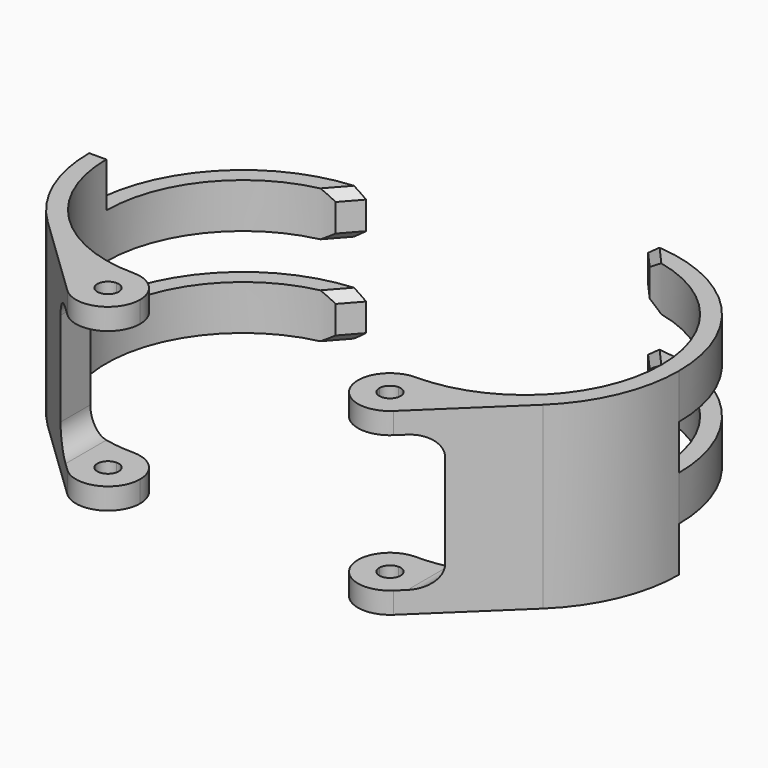
from build123d import *

# Parameters (mm, degrees)
F1_DEPTH      = 21
F2_W          = 90
F2_H          = 32
F3_DEPTH      = 60
F4_R          = 5
F4_2_R        = 5
F5_W          = 36
F5_H          = 10.5
F6_DEPTH      = 80
F7_W          = 36
F7_H          = 10.5
F8_DEPTH      = 80
F9_T1_DEPTH   = 31.1430234422
F9_T3_DEPTH   = 31.1430234422
F9_2_T1_DEPTH = 31.1430234422
F9_2_T3_DEPTH = 31.1430234422
F10_SIZE      = 2
F10_2_SIZE    = 2


# Not quite as in the source:
# - a fillet or chamfer that OpenCascade refuses, or shapes differently, is made with other operations: its cross-section is extruded or revolved along the edge and cut away or added


with BuildPart() as f1:
    # F0 (on Top) → F1 (new body, symmetric)
    with BuildSketch(Plane.XY):
        with BuildLine():
            ThreePointArc((-33, -32), (-65, 0), (-33, 32))
            Line((-33, 32), (-33, 36))
            ThreePointArc((-33, 36), (-66.3997650261, 13.4333799247), (-57.9262073885, -25.9746835443))
            ThreePointArc((-57.9262073885, -25.9746835443), (-49.3189032488, -32.0888360144), (-39.3080154665, -35.4430379747))
            ThreePointArc((-39.3080154665, -35.4430379747), (-36.5932426031, -32.9167935172), (-33, -32))
        make_face()
        with BuildLine():
            Line((-33, -36), (-33, -32))
            ThreePointArc((-33, -32), (-36.5932426031, -32.9167935172), (-39.3080154665, -35.4430379747))
            ThreePointArc((-39.3080154665, -35.4430379747), (-36.166278013, -35.8604891705), (-33, -36))
        make_face()
        with BuildLine():
            ThreePointArc((-26.6919845335, -35.4430379747), (-29.4067573969, -32.9167935172), (-33, -32))
            Line((-33, -32), (-33, -36))
            ThreePointArc((-33, -36), (-29.833721987, -35.8604891705), (-26.6919845335, -35.4430379747))
        make_face()
        with BuildLine():
            ThreePointArc((-25.5, -39.5), (-25.8041638429, -37.3857762652), (-26.6919845335, -35.4430379747))
            ThreePointArc((-26.6919845335, -35.4430379747), (-29.833721987, -35.8604891705), (-33, -36))
            Line((-33, -36), (-33, -37))
            ThreePointArc((-33, -37), (-31.232233047, -37.732233047), (-30.5, -39.5))
            Line((-30.5, -39.5), (-25.5, -39.5))
        make_face()
        with BuildLine():
            ThreePointArc((-38.1929598726, -44.9113924051), (-40.4485261859, -40.3771873561), (-39.3080154665, -35.4430379747))
            ThreePointArc((-39.3080154665, -35.4430379747), (-49.3189032488, -32.0888360144), (-57.9262073885, -25.9746835443))
            Line((-57.9262073885, -25.9746835443), (-38.1929598726, -44.9113924051))
        make_face()
        with BuildLine():
            ThreePointArc((-33, -36), (-36.166278013, -35.8604891705), (-39.3080154665, -35.4430379747))
            ThreePointArc((-39.3080154665, -35.4430379747), (-40.4485261859, -40.3771873561), (-38.1929598726, -44.9113924051))
            ThreePointArc((-38.1929598726, -44.9113924051), (-30.0586736873, -46.399173829), (-25.5, -39.5))
            Line((-25.5, -39.5), (-30.5, -39.5))
            ThreePointArc((-30.5, -39.5), (-34.767766953, -41.267766953), (-33, -37))
            Line((-33, -37), (-33, -36))
        make_face()
    extrude(amount=F1_DEPTH, both=True)


with BuildPart() as f1b:
    # F0 (on Top) → F1, piece 2 (new body, symmetric)
    with BuildSketch(Plane.XY):
        with BuildLine():
            ThreePointArc((69, 0), (58.4558441227, 25.4558441227), (33, 36))
            Line((33, 36), (33, 32))
            ThreePointArc((33, 32), (55.627416998, 22.627416998), (65, 0))
            ThreePointArc((65, 0), (55.627416998, -22.627416998), (33, -32))
            ThreePointArc((33, -32), (36.5932426031, -32.9167935172), (39.3080154665, -35.4430379747))
            ThreePointArc((39.3080154665, -35.4430379747), (49.3189032488, -32.0888360144), (57.9262073885, -25.9746835443))
            ThreePointArc((57.9262073885, -25.9746835443), (66.116034379, -14.1183663009), (69, 0))
        make_face()
        with BuildLine():
            ThreePointArc((33, -32), (29.4067573969, -32.9167935172), (26.6919845335, -35.4430379747))
            ThreePointArc((26.6919845335, -35.4430379747), (29.833721987, -35.8604891705), (33, -36))
            Line((33, -36), (33, -32))
        make_face()
        with BuildLine():
            ThreePointArc((33, -36), (29.833721987, -35.8604891705), (26.6919845335, -35.4430379747))
            ThreePointArc((26.6919845335, -35.4430379747), (25.8041638429, -37.3857762652), (25.5, -39.5))
            Line((25.5, -39.5), (30.5, -39.5))
            ThreePointArc((30.5, -39.5), (31.232233047, -37.732233047), (33, -37))
            Line((33, -37), (33, -36))
        make_face()
        with BuildLine():
            ThreePointArc((39.3080154665, -35.4430379747), (36.5932426031, -32.9167935172), (33, -32))
            Line((33, -32), (33, -36))
            ThreePointArc((33, -36), (36.166278013, -35.8604891705), (39.3080154665, -35.4430379747))
        make_face()
        with BuildLine():
            ThreePointArc((39.3080154665, -35.4430379747), (36.166278013, -35.8604891705), (33, -36))
            Line((33, -36), (33, -37))
            ThreePointArc((33, -37), (34.767766953, -37.732233047), (35.5, -39.5))
            ThreePointArc((35.5, -39.5), (33, -42), (30.5, -39.5))
            Line((30.5, -39.5), (25.5, -39.5))
            ThreePointArc((25.5, -39.5), (30.0586736873, -46.399173829), (38.1929598726, -44.9113924051))
            ThreePointArc((38.1929598726, -44.9113924051), (39.899173829, -42.4413263127), (40.5, -39.5))
            ThreePointArc((40.5, -39.5), (40.1958361571, -37.3857762652), (39.3080154665, -35.4430379747))
        make_face()
        with BuildLine():
            Line((38.1929598726, -44.9113924051), (57.9262073885, -25.9746835443))
            ThreePointArc((57.9262073885, -25.9746835443), (49.3189032488, -32.0888360144), (39.3080154665, -35.4430379747))
            ThreePointArc((39.3080154665, -35.4430379747), (40.1958361571, -37.3857762652), (40.5, -39.5))
            ThreePointArc((40.5, -39.5), (39.899173829, -42.4413263127), (38.1929598726, -44.9113924051))
        make_face()
    extrude(amount=F1_DEPTH, both=True)


with BuildPart() as f3_tool:
    # F2 (on Front) → F3 (new body)
    with BuildSketch(Plane.XZ):
        Rectangle(F2_W, F2_H)
    extrude(amount=F3_DEPTH)


with BuildPart() as f1_1:
    add(f1.part)

    # F3: cut by f3_tool
    add(f3_tool.part, mode=Mode.SUBTRACT)

    # F4
    f4_edges = [f1_1.edges().sort_by_distance(p)[0] for p in [
        (-45, -34.021957, 16),
        (-45, -34.021957, -16),
    ]]
    fillet(f4_edges, radius=F4_R)

    # F5 (on Right) → F6 (cut)
    with BuildSketch(Plane.YZ):
        with Locations((18, 15.75)):
            Rectangle(F5_W, F5_H)
        with Locations((18, -5.25)):
            Rectangle(F5_W, F5_H)
    extrude(amount=-F6_DEPTH, mode=Mode.SUBTRACT)

    # F9: chamfer of 4.25 on 2 edges, made by hand

    # F9_s2 → F9_t1 (cut)
    with BuildSketch(Plane.XY.offset(-10.3215117211)):
        with BuildLine():
            Line((-36.7517241379, 31.7793103448), (-33, 36))
            Line((-33, 36), (-33, 32))
            ThreePointArc((-33, 32), (-34.9393186322, 31.9411809932), (-36.7517241379, 31.7793103448))
        make_face()
    extrude(amount=F9_T1_DEPTH, mode=Mode.SUBTRACT)

    # F9_s4 → F9_t3 (cut)
    with BuildSketch(Plane.XY.offset(-31.3215117211)):
        with BuildLine():
            Line((-36.7517241379, 31.7793103448), (-33, 36))
            Line((-33, 36), (-33, 32))
            ThreePointArc((-33, 32), (-34.9393186322, 31.9411809932), (-36.7517241379, 31.7793103448))
        make_face()
    extrude(amount=F9_T3_DEPTH, mode=Mode.SUBTRACT)

    # F10
    f10_edges = [f1_1.edges().sort_by_distance(p)[0] for p in [
        (-34.875862, 33.889655, 10.5),
        (-34.875862, 33.889655, -10.5),
        (-34.875862, 33.889655, -21),
        (-34.875862, 33.889655, 0),
    ]]
    chamfer(f10_edges, length=F10_SIZE)


with BuildPart() as f1b_1:
    add(f1b.part)

    # F3: cut by f3_tool
    add(f3_tool.part, mode=Mode.SUBTRACT)

    # F4#2
    f4_2_edges = [f1b_1.edges().sort_by_distance(p)[0] for p in [
        (45, -34.021957, 16),
        (45, -34.021957, -16),
    ]]
    fillet(f4_2_edges, radius=F4_2_R)

    # F7 (on Right) → F8 (cut)
    with BuildSketch(Plane.YZ):
        with Locations((18, 5.25)):
            Rectangle(F7_W, F7_H)
        with Locations((18, -15.75)):
            Rectangle(F7_W, F7_H)
    extrude(amount=F8_DEPTH, mode=Mode.SUBTRACT)

    # F9#2: chamfer of 4.25 on 2 edges, made by hand

    # F9_2_s2 → F9_2_t1 (cut)
    with BuildSketch(Plane.XY.offset(0.1784882789)):
        with BuildLine():
            Line((36.7517241379, 31.7793103448), (33, 36))
            Line((33, 36), (33, 32))
            ThreePointArc((33, 32), (34.9393186322, 31.9411809932), (36.7517241379, 31.7793103448))
        make_face()
    extrude(amount=F9_2_T1_DEPTH, mode=Mode.SUBTRACT)

    # F9_2_s4 → F9_2_t3 (cut)
    with BuildSketch(Plane.XY.offset(-20.8215117211)):
        with BuildLine():
            Line((36.7517241379, 31.7793103448), (33, 36))
            Line((33, 36), (33, 32))
            ThreePointArc((33, 32), (34.9393186322, 31.9411809932), (36.7517241379, 31.7793103448))
        make_face()
    extrude(amount=F9_2_T3_DEPTH, mode=Mode.SUBTRACT)

    # F10#2
    f10_2_edges = [f1b_1.edges().sort_by_distance(p)[0] for p in [
        (34.875862, 33.889655, -10.5),
        (34.875862, 33.889655, 10.5),
        (34.875862, 33.889655, 21),
        (34.875862, 33.889655, 0),
    ]]
    chamfer(f10_2_edges, length=F10_2_SIZE)


solid = Compound([f1_1.part, f1b_1.part])
